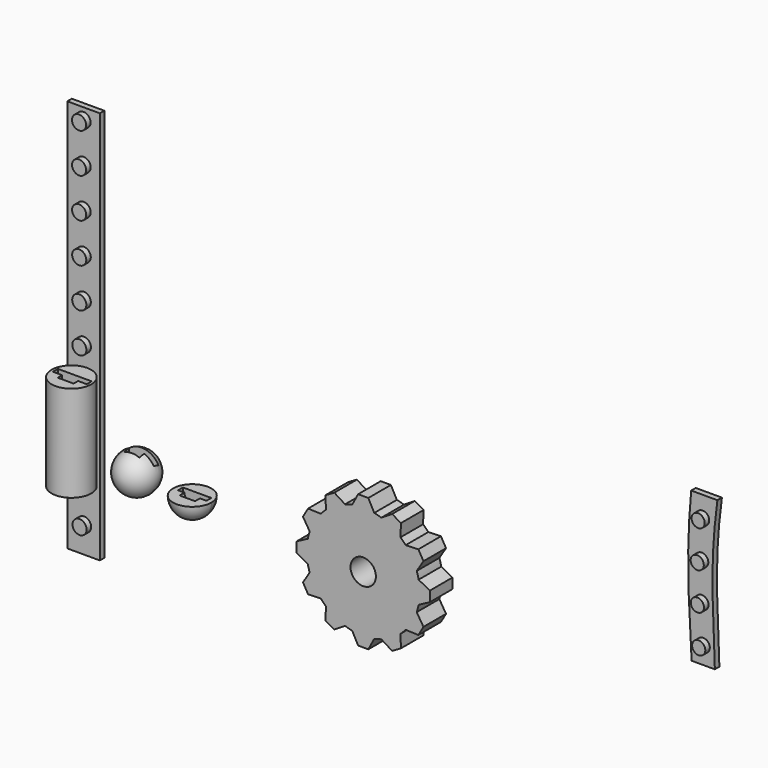
from build123d import *

# Parameters (mm, degrees)
F1_DEPTH       = 6.35
F0_R           = 2.8524956038
F2_DEPTH       = 6.35
F0_R_2         = 1.4795803684
F3_DEPTH       = 2.54
F4_DEPTH       = 1.27
F0_W           = 7.3252171278
F0_H           = 88.480938226
F0_R_3         = 1.5875
F5_DEPTH       = 1.27
F6_DEPTH       = 2.54
F7_R           = 4.445
F8_DEPTH       = 21.59
F9_ANGLE       = 180
F11_DEPTH      = 25.4
F11_DEPTH_BACK = 25.4


# Not quite as in the source:
# - a feature names something its author has since deleted; it is built from what else it names


with BuildPart() as f1:
    # F0 (on Front) → F1 (new body)
    with BuildSketch(Plane.XZ):
        with BuildLine():
            Line((12.3960816659, 8.4804374198), (9.543899784, 8.3787813501))
            ThreePointArc((9.543899784, 8.3787813501), (10.9985226281, 6.35), (12.0281873939, 4.0758689891))
            Line((12.0281873939, 4.0758689891), (13.5423150737, 6.4951029202))
            Line((13.5423150737, 6.4951029202), (12.3960816659, 8.4804374198))
        make_face()
    extrude(amount=F1_DEPTH)


with BuildPart() as f1b:
    # F0 (on Front) → F1, piece 2 (new body)
    with BuildSketch(Plane.XZ):
        with BuildLine():
            Line((6.4951029202, 13.5423150737), (4.0758689891, 12.0281873939))
            ThreePointArc((4.0758689891, 12.0281873939), (6.35, 10.9985226281), (8.3787813501, 9.543899784))
            Line((8.3787813501, 9.543899784), (8.4804374198, 12.3960816659))
            Line((8.4804374198, 12.3960816659), (6.4951029202, 13.5423150737))
        make_face()
    extrude(amount=F1_DEPTH)


with BuildPart() as f1c:
    # F0 (on Front) → F1, piece 3 (new body)
    with BuildSketch(Plane.XZ):
        with BuildLine():
            ThreePointArc((-12.0281873939, 4.0758689891), (-10.9985226281, 6.35), (-9.543899784, 8.3787813501))
            Line((-9.543899784, 8.3787813501), (-12.3960816659, 8.4804374198))
            Line((-12.3960816659, 8.4804374198), (-13.5423150737, 6.4951029202))
            Line((-13.5423150737, 6.4951029202), (-12.0281873939, 4.0758689891))
        make_face()
    extrude(amount=F1_DEPTH)


with BuildPart() as f1d:
    # F0 (on Front) → F1, piece 4 (new body)
    with BuildSketch(Plane.XZ):
        with BuildLine():
            ThreePointArc((-12.4546503392, -2.4842876099), (-12.7, 0), (-12.4546503392, 2.4842876099))
            Line((-12.4546503392, 2.4842876099), (-14.9755403399, 1.1462334078))
            Line((-14.9755403399, 1.1462334078), (-14.9755403399, -1.1462334078))
            Line((-14.9755403399, -1.1462334078), (-12.4546503392, -2.4842876099))
        make_face()
    extrude(amount=F1_DEPTH)


with BuildPart() as f1e:
    # F0 (on Front) → F1, piece 5 (new body)
    with BuildSketch(Plane.XZ):
        with BuildLine():
            ThreePointArc((-9.543899784, -8.3787813501), (-10.9985226281, -6.35), (-12.0281873939, -4.0758689891))
            Line((-12.0281873939, -4.0758689891), (-13.5423150737, -6.4951029202))
            Line((-13.5423150737, -6.4951029202), (-12.3960816659, -8.4804374198))
            Line((-12.3960816659, -8.4804374198), (-9.543899784, -8.3787813501))
        make_face()
    extrude(amount=F1_DEPTH)


with BuildPart() as f1f:
    # F0 (on Front) → F1, piece 6 (new body)
    with BuildSketch(Plane.XZ):
        with BuildLine():
            ThreePointArc((-4.0758689891, -12.0281873939), (-6.35, -10.9985226281), (-8.3787813501, -9.543899784))
            Line((-8.3787813501, -9.543899784), (-8.4804374198, -12.3960816659))
            Line((-8.4804374198, -12.3960816659), (-6.4951029202, -13.5423150737))
            Line((-6.4951029202, -13.5423150737), (-4.0758689891, -12.0281873939))
        make_face()
    extrude(amount=F1_DEPTH)


with BuildPart() as f1g:
    # F0 (on Front) → F1, piece 7 (new body)
    with BuildSketch(Plane.XZ):
        with BuildLine():
            Line((1.1462334078, -14.9755403399), (2.4842876099, -12.4546503392))
            ThreePointArc((2.4842876099, -12.4546503392), (0, -12.7), (-2.4842876099, -12.4546503392))
            Line((-2.4842876099, -12.4546503392), (-1.1462334078, -14.9755403399))
            Line((-1.1462334078, -14.9755403399), (1.1462334078, -14.9755403399))
        make_face()
    extrude(amount=F1_DEPTH)


with BuildPart() as f1h:
    # F0 (on Front) → F1, piece 8 (new body)
    with BuildSketch(Plane.XZ):
        with BuildLine():
            Line((8.4804374198, -12.3960816659), (8.3787813501, -9.543899784))
            ThreePointArc((8.3787813501, -9.543899784), (6.35, -10.9985226281), (4.0758689891, -12.0281873939))
            Line((4.0758689891, -12.0281873939), (6.4951029202, -13.5423150737))
            Line((6.4951029202, -13.5423150737), (8.4804374198, -12.3960816659))
        make_face()
    extrude(amount=F1_DEPTH)


with BuildPart() as f1i:
    # F0 (on Front) → F1, piece 9 (new body)
    with BuildSketch(Plane.XZ):
        with BuildLine():
            Line((13.5423150737, -6.4951029202), (12.0281873939, -4.0758689891))
            ThreePointArc((12.0281873939, -4.0758689891), (10.9985226281, -6.35), (9.543899784, -8.3787813501))
            Line((9.543899784, -8.3787813501), (12.3960816659, -8.4804374198))
            Line((12.3960816659, -8.4804374198), (13.5423150737, -6.4951029202))
        make_face()
    extrude(amount=F1_DEPTH)


with BuildPart() as f1j:
    # F0 (on Front) → F1, piece 10 (new body)
    with BuildSketch(Plane.XZ):
        with BuildLine():
            Line((14.9755403399, 1.1462334078), (12.4546503392, 2.4842876099))
            ThreePointArc((12.4546503392, 2.4842876099), (12.6385137439, 1.2481868234), (12.7, 0))
            ThreePointArc((12.7, 0), (12.6385137439, -1.2481868234), (12.4546503392, -2.4842876099))
            Line((12.4546503392, -2.4842876099), (14.9755403399, -1.1462334078))
            Line((14.9755403399, -1.1462334078), (14.9755403399, 1.1462334078))
        make_face()
    extrude(amount=F1_DEPTH)


with BuildPart() as f1k:
    # F0 (on Front) → F1, piece 11 (new body)
    with BuildSketch(Plane.XZ):
        with BuildLine():
            Line((2.4842876099, 12.4546503392), (1.1462334078, 14.9755403399))
            Line((1.1462334078, 14.9755403399), (-1.1462334078, 14.9755403399))
            Line((-1.1462334078, 14.9755403399), (-2.4842876099, 12.4546503392))
            ThreePointArc((-2.4842876099, 12.4546503392), (0, 12.7), (2.4842876099, 12.4546503392))
        make_face()
    extrude(amount=F1_DEPTH)


with BuildPart() as f1l:
    # F0 (on Front) → F1, piece 12 (new body)
    with BuildSketch(Plane.XZ):
        with BuildLine():
            ThreePointArc((-8.3787813501, 9.543899784), (-6.35, 10.9985226281), (-4.0758689891, 12.0281873939))
            Line((-4.0758689891, 12.0281873939), (-6.4951029202, 13.5423150737))
            Line((-6.4951029202, 13.5423150737), (-8.4804374198, 12.3960816659))
            Line((-8.4804374198, 12.3960816659), (-8.3787813501, 9.543899784))
        make_face()
    extrude(amount=F1_DEPTH)


with BuildPart() as f2:
    # F0 (on Front) → F2 (new body)
    with BuildSketch(Plane.XZ):
        with BuildLine():
            Line((2.4842876099, 12.4546503392), (1.1462334078, 14.9755403399))
            Line((1.1462334078, 14.9755403399), (-1.1462334078, 14.9755403399))
            Line((-1.1462334078, 14.9755403399), (-2.4842876099, 12.4546503392))
            ThreePointArc((-2.4842876099, 12.4546503392), (0, 12.7), (2.4842876099, 12.4546503392))
        make_face()
        with BuildLine():
            Line((12.3960816659, 8.4804374198), (9.543899784, 8.3787813501))
            ThreePointArc((9.543899784, 8.3787813501), (10.9985226281, 6.35), (12.0281873939, 4.0758689891))
            Line((12.0281873939, 4.0758689891), (13.5423150737, 6.4951029202))
            Line((13.5423150737, 6.4951029202), (12.3960816659, 8.4804374198))
        make_face()
        with BuildLine():
            Line((6.4951029202, 13.5423150737), (4.0758689891, 12.0281873939))
            ThreePointArc((4.0758689891, 12.0281873939), (6.35, 10.9985226281), (8.3787813501, 9.543899784))
            Line((8.3787813501, 9.543899784), (8.4804374198, 12.3960816659))
            Line((8.4804374198, 12.3960816659), (6.4951029202, 13.5423150737))
        make_face()
        with BuildLine():
            ThreePointArc((-8.3787813501, 9.543899784), (-6.35, 10.9985226281), (-4.0758689891, 12.0281873939))
            Line((-4.0758689891, 12.0281873939), (-6.4951029202, 13.5423150737))
            Line((-6.4951029202, 13.5423150737), (-8.4804374198, 12.3960816659))
            Line((-8.4804374198, 12.3960816659), (-8.3787813501, 9.543899784))
        make_face()
        with BuildLine():
            ThreePointArc((-12.0281873939, 4.0758689891), (-10.9985226281, 6.35), (-9.543899784, 8.3787813501))
            Line((-9.543899784, 8.3787813501), (-12.3960816659, 8.4804374198))
            Line((-12.3960816659, 8.4804374198), (-13.5423150737, 6.4951029202))
            Line((-13.5423150737, 6.4951029202), (-12.0281873939, 4.0758689891))
        make_face()
        with BuildLine():
            ThreePointArc((-12.4546503392, -2.4842876099), (-12.7, 0), (-12.4546503392, 2.4842876099))
            Line((-12.4546503392, 2.4842876099), (-14.9755403399, 1.1462334078))
            Line((-14.9755403399, 1.1462334078), (-14.9755403399, -1.1462334078))
            Line((-14.9755403399, -1.1462334078), (-12.4546503392, -2.4842876099))
        make_face()
        with BuildLine():
            ThreePointArc((-9.543899784, -8.3787813501), (-10.9985226281, -6.35), (-12.0281873939, -4.0758689891))
            Line((-12.0281873939, -4.0758689891), (-13.5423150737, -6.4951029202))
            Line((-13.5423150737, -6.4951029202), (-12.3960816659, -8.4804374198))
            Line((-12.3960816659, -8.4804374198), (-9.543899784, -8.3787813501))
        make_face()
        with BuildLine():
            ThreePointArc((-4.0758689891, -12.0281873939), (-6.35, -10.9985226281), (-8.3787813501, -9.543899784))
            Line((-8.3787813501, -9.543899784), (-8.4804374198, -12.3960816659))
            Line((-8.4804374198, -12.3960816659), (-6.4951029202, -13.5423150737))
            Line((-6.4951029202, -13.5423150737), (-4.0758689891, -12.0281873939))
        make_face()
        with BuildLine():
            Line((1.1462334078, -14.9755403399), (2.4842876099, -12.4546503392))
            ThreePointArc((2.4842876099, -12.4546503392), (0, -12.7), (-2.4842876099, -12.4546503392))
            Line((-2.4842876099, -12.4546503392), (-1.1462334078, -14.9755403399))
            Line((-1.1462334078, -14.9755403399), (1.1462334078, -14.9755403399))
        make_face()
        with BuildLine():
            Line((8.4804374198, -12.3960816659), (8.3787813501, -9.543899784))
            ThreePointArc((8.3787813501, -9.543899784), (6.35, -10.9985226281), (4.0758689891, -12.0281873939))
            Line((4.0758689891, -12.0281873939), (6.4951029202, -13.5423150737))
            Line((6.4951029202, -13.5423150737), (8.4804374198, -12.3960816659))
        make_face()
        with BuildLine():
            Line((13.5423150737, -6.4951029202), (12.0281873939, -4.0758689891))
            ThreePointArc((12.0281873939, -4.0758689891), (10.9985226281, -6.35), (9.543899784, -8.3787813501))
            Line((9.543899784, -8.3787813501), (12.3960816659, -8.4804374198))
            Line((12.3960816659, -8.4804374198), (13.5423150737, -6.4951029202))
        make_face()
        with BuildLine():
            Line((14.9755403399, 1.1462334078), (12.4546503392, 2.4842876099))
            ThreePointArc((12.4546503392, 2.4842876099), (12.6385137439, 1.2481868234), (12.7, 0))
            ThreePointArc((12.7, 0), (12.6385137439, -1.2481868234), (12.4546503392, -2.4842876099))
            Line((12.4546503392, -2.4842876099), (14.9755403399, -1.1462334078))
            Line((14.9755403399, -1.1462334078), (14.9755403399, 1.1462334078))
        make_face()
        with BuildLine():
            ThreePointArc((4.0758689891, 12.0281873939), (3.2870018728, 12.2672579939), (2.4842876099, 12.4546503392))
            ThreePointArc((2.4842876099, 12.4546503392), (0, 12.7), (-2.4842876099, 12.4546503392))
            ThreePointArc((-2.4842876099, 12.4546503392), (-3.2870018728, 12.2672579939), (-4.0758689891, 12.0281873939))
            ThreePointArc((-4.0758689891, 12.0281873939), (-6.35, 10.9985226281), (-8.3787813501, 9.543899784))
            ThreePointArc((-8.3787813501, 9.543899784), (-8.9802561211, 8.9802561211), (-9.543899784, 8.3787813501))
            ThreePointArc((-9.543899784, 8.3787813501), (-10.9985226281, 6.35), (-12.0281873939, 4.0758689891))
            ThreePointArc((-12.0281873939, 4.0758689891), (-12.2672579939, 3.2870018728), (-12.4546503392, 2.4842876099))
            ThreePointArc((-12.4546503392, 2.4842876099), (-12.7, 0), (-12.4546503392, -2.4842876099))
            ThreePointArc((-12.4546503392, -2.4842876099), (-12.2672579939, -3.2870018728), (-12.0281873939, -4.0758689891))
            ThreePointArc((-12.0281873939, -4.0758689891), (-10.9985226281, -6.35), (-9.543899784, -8.3787813501))
            ThreePointArc((-9.543899784, -8.3787813501), (-8.9802561211, -8.9802561211), (-8.3787813501, -9.543899784))
            ThreePointArc((-8.3787813501, -9.543899784), (-6.35, -10.9985226281), (-4.0758689891, -12.0281873939))
            ThreePointArc((-4.0758689891, -12.0281873939), (-3.2870018728, -12.2672579939), (-2.4842876099, -12.4546503392))
            ThreePointArc((-2.4842876099, -12.4546503392), (0, -12.7), (2.4842876099, -12.4546503392))
            ThreePointArc((2.4842876099, -12.4546503392), (3.2870018728, -12.2672579939), (4.0758689891, -12.0281873939))
            ThreePointArc((4.0758689891, -12.0281873939), (6.35, -10.9985226281), (8.3787813501, -9.543899784))
            ThreePointArc((8.3787813501, -9.543899784), (8.9802561211, -8.9802561211), (9.543899784, -8.3787813501))
            ThreePointArc((9.543899784, -8.3787813501), (10.9985226281, -6.35), (12.0281873939, -4.0758689891))
            ThreePointArc((12.0281873939, -4.0758689891), (12.2672579939, -3.2870018728), (12.4546503392, -2.4842876099))
            ThreePointArc((12.4546503392, -2.4842876099), (12.6385137439, -1.2481868234), (12.7, 0))
            ThreePointArc((12.7, 0), (12.6385137439, 1.2481868234), (12.4546503392, 2.4842876099))
            ThreePointArc((12.4546503392, 2.4842876099), (12.2672579939, 3.2870018728), (12.0281873939, 4.0758689891))
            ThreePointArc((12.0281873939, 4.0758689891), (10.9985226281, 6.35), (9.543899784, 8.3787813501))
            ThreePointArc((9.543899784, 8.3787813501), (8.9802561211, 8.9802561211), (8.3787813501, 9.543899784))
            ThreePointArc((8.3787813501, 9.543899784), (6.35, 10.9985226281), (4.0758689891, 12.0281873939))
        make_face()
        Circle(F0_R, mode=Mode.SUBTRACT)
    extrude(amount=F2_DEPTH)


with BuildPart() as f3:
    # F0 (on Front) → F3 (new body)
    with BuildSketch(Plane.XZ):
        with Locations((72.2401882558, 32.066884822)):
            Circle(F0_R_2)
    extrude(amount=F3_DEPTH)


with BuildPart() as f3b:
    # F0 (on Front) → F3, piece 2 (new body)
    with BuildSketch(Plane.XZ):
        with Locations((72.0286418181, 23.6875547709)):
            Circle(F0_R_2)
    extrude(amount=F3_DEPTH)


with BuildPart() as f3c:
    # F0 (on Front) → F3, piece 3 (new body)
    with BuildSketch(Plane.XZ):
        with Locations((72.0710953803, 15.3082247199)):
            Circle(F0_R_2)
    extrude(amount=F3_DEPTH)


with BuildPart() as f3d:
    # F0 (on Front) → F3, piece 4 (new body)
    with BuildSketch(Plane.XZ):
        with Locations((72.3675489426, 6.9288946688)):
            Circle(F0_R_2)
    extrude(amount=F3_DEPTH)


with BuildPart() as f4:
    # F0 (on Front) → F4 (new body)
    with BuildSketch(Plane.XZ):
        with BuildLine():
            add(Edge.make_bspline(
                [(69.7565302253, 3.0123661272), (69.2636471486, 11.1810116625), (68.5910347248, 22.3698418828), (69.3795084682, 33.631622489), (69.6598606342, 36.6658026495)],
                knots=[0, 0, 0, 0, 0.4992578952, 0.6838997793, 0.6838997793, 0.6838997793, 0.6838997793], degree=3))
            Line((69.7565302253, 3.0123661272), (74.9785676599, 3.0123661272))
            add(Edge.make_bspline(
                [(74.9785676599, 3.0123661272), (74.7175919308, 11.1681350458), (73.8946936347, 22.3825032061), (75.1632531485, 33.6326874012), (75.5508983315, 36.6658026495)],
                knots=[0, 0, 0, 0, 0.4990456515, 0.6838015307, 0.6838015307, 0.6838015307, 0.6838015307], degree=3))
            Line((75.5508983315, 36.6658026495), (69.6598606342, 36.6658026495))
        make_face()
        with Locations((72.3675489426, 6.9288946688)):
            Circle(F0_R_2, mode=Mode.SUBTRACT)
        with Locations((72.0710953803, 15.3082247199)):
            Circle(F0_R_2, mode=Mode.SUBTRACT)
        with Locations((72.0286418181, 23.6875547709)):
            Circle(F0_R_2, mode=Mode.SUBTRACT)
        with Locations((72.2401882558, 32.066884822)):
            Circle(F0_R_2, mode=Mode.SUBTRACT)
    extrude(amount=F4_DEPTH)


with BuildPart() as f5:
    # F0 (on Front) → F5 (new body)
    with BuildSketch(Plane.XZ):
        with Locations((-66.9246315956, 23.8421093673)):
            Rectangle(F0_W, F0_H)
        with Locations((-66.8016991951, -14.4197772568)):
            Circle(F0_R_3, mode=Mode.SUBTRACT)
        with Locations((-66.8153583508, -5.5297877502)):
            Circle(F0_R_3, mode=Mode.SUBTRACT)
        with Locations((-66.8290175064, 3.3602017564)):
            Circle(F0_R_3, mode=Mode.SUBTRACT)
        with Locations((-66.842676662, 12.250191263)):
            Circle(F0_R_3, mode=Mode.SUBTRACT)
        with Locations((-66.8563358176, 21.1401807696)):
            Circle(F0_R_3, mode=Mode.SUBTRACT)
        with Locations((-66.8699949732, 30.0301702762)):
            Circle(F0_R_3, mode=Mode.SUBTRACT)
        with Locations((-66.8836541288, 38.9201597828)):
            Circle(F0_R_3, mode=Mode.SUBTRACT)
        with Locations((-66.8973132844, 47.8101492894)):
            Circle(F0_R_3, mode=Mode.SUBTRACT)
        with Locations((-66.91097244, 56.700138796)):
            Circle(F0_R_3, mode=Mode.SUBTRACT)
        with Locations((-66.9246315956, 65.5901283026)):
            Circle(F0_R_3, mode=Mode.SUBTRACT)
    extrude(amount=F5_DEPTH)


with BuildPart() as f6:
    # F0 (on Front) → F6 (new body)
    with BuildSketch(Plane.XZ):
        with Locations((-66.9246315956, 65.5901283026)):
            Circle(F0_R_3)
    extrude(amount=F6_DEPTH)


with BuildPart() as f6b:
    # F0 (on Front) → F6, piece 2 (new body)
    with BuildSketch(Plane.XZ):
        with Locations((-66.91097244, 56.700138796)):
            Circle(F0_R_3)
    extrude(amount=F6_DEPTH)


with BuildPart() as f6c:
    # F0 (on Front) → F6, piece 3 (new body)
    with BuildSketch(Plane.XZ):
        with Locations((-66.8973132844, 47.8101492894)):
            Circle(F0_R_3)
    extrude(amount=F6_DEPTH)


with BuildPart() as f6d:
    # F0 (on Front) → F6, piece 4 (new body)
    with BuildSketch(Plane.XZ):
        with Locations((-66.8836541288, 38.9201597828)):
            Circle(F0_R_3)
    extrude(amount=F6_DEPTH)


with BuildPart() as f6e:
    # F0 (on Front) → F6, piece 5 (new body)
    with BuildSketch(Plane.XZ):
        with Locations((-66.8699949732, 30.0301702762)):
            Circle(F0_R_3)
    extrude(amount=F6_DEPTH)


with BuildPart() as f6f:
    # F0 (on Front) → F6, piece 6 (new body)
    with BuildSketch(Plane.XZ):
        with Locations((-66.8563358176, 21.1401807696)):
            Circle(F0_R_3)
    extrude(amount=F6_DEPTH)


with BuildPart() as f6g:
    # F0 (on Front) → F6, piece 7 (new body)
    with BuildSketch(Plane.XZ):
        with Locations((-66.842676662, 12.250191263)):
            Circle(F0_R_3)
    extrude(amount=F6_DEPTH)


with BuildPart() as f6h:
    # F0 (on Front) → F6, piece 8 (new body)
    with BuildSketch(Plane.XZ):
        with Locations((-66.8290175064, 3.3602017564)):
            Circle(F0_R_3)
    extrude(amount=F6_DEPTH)


with BuildPart() as f6i:
    # F0 (on Front) → F6, piece 9 (new body)
    with BuildSketch(Plane.XZ):
        with Locations((-66.8016991951, -14.4197772568)):
            Circle(F0_R_3)
    extrude(amount=F6_DEPTH)


with BuildPart() as f6j:
    # F0 (on Front) → F6, piece 10 (new body)
    with BuildSketch(Plane.XZ):
        with Locations((-66.8153583508, -5.5297877502)):
            Circle(F0_R_3)
    extrude(amount=F6_DEPTH)


with BuildPart() as f8:
    # F7 (on Top) → F8 (new body)
    with BuildSketch(Plane.XY):
        with Locations((-60.3255299519, -12.9298945169)):
            Circle(F7_R)
        Polygon((-64.1300623113, -13.3871221616), (-64.1300623113, -11.9780084066), (-56.5209975925, -11.9780084066), (-56.5209975925, -13.3686087251), (-58.4649176252, -13.3686087251), (-58.4649176252, -14.6275295365), (-62.0380274302, -14.6275295365), (-62.0380274302, -13.3871221616), align=None, mode=Mode.SUBTRACT)
    extrude(amount=F8_DEPTH)


with BuildPart() as f9:
    # F7 (on Top) → F9 (revolve)
    with BuildSketch(Plane.XY):
        with BuildLine():
            Line((-41.54393715, 1.8545307278), (-41.54393715, -1.0930870515))
            Line((-41.54393715, -1.0930870515), (-38.3533991345, -1.0930870515))
            Line((-38.3533991345, -1.0930870515), (-38.3533991345, -2.4659501158))
            Line((-38.3533991345, -2.4659501158), (-39.8073117004, -2.4659501158))
            Line((-39.8073117004, -2.4659501158), (-39.8073117004, -3.8388130651))
            Line((-39.8073117004, -3.8388130651), (-41.54393715, -3.8388130651))
            Line((-41.54393715, -3.8388130651), (-41.54393715, -6.7618094404))
            ThreePointArc((-41.54393715, -6.7618094404), (-38.497600869, -5.4999756373), (-37.2357670659, -2.4536393563))
            ThreePointArc((-37.2357670659, -2.4536393563), (-38.497600869, 0.5926969246), (-41.54393715, 1.8545307278))
        make_face()
    revolve(axis=Axis((-41.54393715, -2.4536393563, 0), (0, 1, 0)), revolution_arc=F9_ANGLE)


with BuildPart() as f10:
    # F7 (on Top) → F10 (revolve)
    with BuildSketch(Plane.XY):
        with BuildLine():
            Line((-58.5492192088, -0.2415674766), (-54.7070381038, -0.2415674766))
            Line((-54.7070381038, -0.2415674766), (-54.7070381038, 2.9141384635))
            ThreePointArc((-54.7070381038, 2.9141384635), (-59.2210538461, -1.5998772788), (-54.7070381038, -6.1138930211))
            Line((-54.7070381038, -6.1138930211), (-54.7070381038, -2.958187081))
            Line((-54.7070381038, -2.958187081), (-56.4116651521, -2.958187081))
            Line((-56.4116651521, -2.958187081), (-56.4116651521, -1.5782490663))
            Line((-56.4116651521, -1.5782490663), (-58.5492192088, -1.5782490663))
            Line((-58.5492192088, -1.5782490663), (-58.5492192088, -0.2415674766))
        make_face()
        Polygon((-54.7070381038, -2.958187081), (-54.7070381038, -0.2415674766), (-58.5492192088, -0.2415674766), (-58.5492192088, -1.5782490663), (-56.4116651521, -1.5782490663), (-56.4116651521, -2.958187081), align=None)
    revolve(axis=Axis((-54.7070381038, -1.5998772788, 0), (0, -1, 0)))

    # F7 (on Top) → F11 (cut, two sides)
    with BuildSketch(Plane.XY) as f11_sk:
        Polygon((-50.8648569988, -0.2415674766), (-54.7070381038, -0.2415674766), (-54.7070381038, -2.958187081), (-53.0024110555, -2.958187081), (-53.0024110555, -1.5782490663), (-50.8648569988, -1.5782490663), align=None)
        Polygon((-54.7070381038, -2.958187081), (-54.7070381038, -0.2415674766), (-58.5492192088, -0.2415674766), (-58.5492192088, -1.5782490663), (-56.4116651521, -1.5782490663), (-56.4116651521, -2.958187081), align=None)
    extrude(amount=-F11_DEPTH, mode=Mode.SUBTRACT)
    extrude(f11_sk.sketch, amount=F11_DEPTH_BACK, mode=Mode.SUBTRACT)


solid = Compound([f1.part, f1b.part, f1c.part, f1d.part, f1e.part, f1f.part, f1g.part, f1h.part, f1i.part, f1j.part, f1k.part, f1l.part, f2.part, f3.part, f3b.part, f3c.part, f3d.part, f4.part, f5.part, f6.part, f6b.part, f6c.part, f6d.part, f6e.part, f6f.part, f6g.part, f6h.part, f6i.part, f6j.part, f8.part, f9.part, f10.part])
